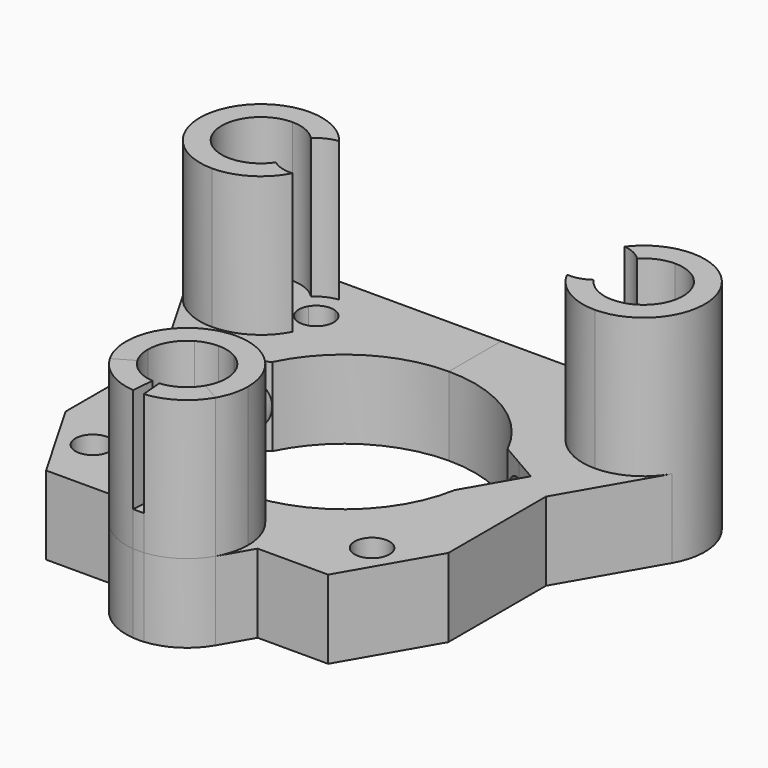
from build123d import *
from build123d import SkipClean  # not in build123d's __all__

# Parameters (mm, degrees)
F0_R     = 2
F1_DEPTH = 9
F2_DEPTH = 25
F4_DEPTH = 25
F6_DEPTH = 13


with BuildPart() as f1:
    # F0 (on Top) → F1 (new body)
    with BuildSketch(Plane.XY):
        with BuildLine():
            Line((-28.0014880557, 34.5), (-21.9393102292, 24))
            Line((-21.9393102292, 24), (-21.9393102292, 31))
            ThreePointArc((-21.9393102292, 31), (-25.4393102292, 31.9378221735), (-28.0014880557, 34.5))
        make_face()
        with BuildLine():
            Line((0, 4.5), (0, 7))
            ThreePointArc((0, 7), (-1.8117333157, 6.761480784), (-3.5, 6.0621778265))
            Line((-3.5, 6.0621778265), (-2.25, 3.897114317))
            ThreePointArc((-2.25, 3.897114317), (-1.164685703, 4.3466662183), (0, 4.5))
        make_face()
        with BuildLine():
            Line((-19.6893102292, 34.102885683), (-18.4393102292, 31.9378221735))
            ThreePointArc((-18.4393102292, 31.9378221735), (-16.8860218217, 33.1560061653), (-15.7345912365, 34.759404033))
            ThreePointArc((-15.7345912365, 34.759404033), (-17.0382696465, 34.8965993643), (-18.2150742777, 35.4741206329))
            ThreePointArc((-18.2150742777, 35.4741206329), (-18.8745190254, 34.7049954663), (-19.6893102292, 34.102885683))
        make_face()
        with BuildLine():
            Line((-3.5, 6.0621778265), (-4.7820020843, 8.282670572))
            ThreePointArc((-4.7820020843, 8.282670572), (-9.4997383801, 10.8915991321), (-12.9903810568, 15))
            Line((-12.9903810568, 15), (-15.8049636191, 13.375))
            Line((-15.8049636191, 13.375), (-8.0829037687, 0))
            Line((-8.0829037687, 0), (-7, 0))
            ThreePointArc((-7, 0), (-6.0621778265, 3.5), (-3.5, 6.0621778265))
        make_face()
        with BuildLine():
            Line((-21.9393102292, 38), (-21.9393102292, 42.5))
            ThreePointArc((-21.9393102292, 42.5), (-25.8364245462, 40.25), (-25.8364245462, 35.75))
            Line((-25.8364245462, 35.75), (-21.9393102292, 38))
        make_face()
        with BuildLine():
            Line((-2.25, 3.897114317), (-3.5, 6.0621778265))
            ThreePointArc((-3.5, 6.0621778265), (-6.0621778265, 3.5), (-7, 0))
            Line((-7, 0), (-4.5, 0))
            ThreePointArc((-4.5, 0), (-3.897114317, 2.25), (-2.25, 3.897114317))
        make_face()
        with BuildLine():
            ThreePointArc((-18.2150742777, 35.4741206329), (-17.0382696465, 34.8965993643), (-15.7345912365, 34.759404033))
            ThreePointArc((-15.7345912365, 34.759404033), (-15.3199791984, 35.7230597934), (-15.0540367364, 36.7378554248))
            ThreePointArc((-15.0540367364, 36.7378554248), (-16.3628996791, 36.5331995976), (-17.5125398242, 37.1914805006))
            ThreePointArc((-17.5125398242, 37.1914805006), (-17.7743303511, 36.296197601), (-18.2150742777, 35.4741206329))
        make_face()
        with BuildLine():
            Line((-21.9393102292, 33.5), (-21.9393102292, 38))
            Line((-21.9393102292, 38), (-25.8364245462, 35.75))
            ThreePointArc((-25.8364245462, 35.75), (-24.1893102292, 34.102885683), (-21.9393102292, 33.5))
        make_face()
        with BuildLine():
            ThreePointArc((7, 0), (4.9497474683, 4.9497474683), (0, 7))
            Line((0, 7), (0, 4.5))
            ThreePointArc((0, 4.5), (3.1819805153, 3.1819805153), (4.5, 0))
            ThreePointArc((4.5, 0), (3.3177480156, -3.0401559343), (0.3922008424, -4.4828761414))
            Line((0.3922008424, -4.4828761414), (0.6100901992, -6.9733628866))
            ThreePointArc((0.6100901992, -6.9733628866), (5.1609413577, -4.7291314533), (7, 0))
        make_face()
        with BuildLine():
            Line((-4.5, 0), (-7, 0))
            ThreePointArc((-7, 0), (-6.761480784, -1.8117333157), (-6.0621778265, -3.5))
            Line((-6.0621778265, -3.5), (-3.897114317, -2.25))
            ThreePointArc((-3.897114317, -2.25), (-4.3466662183, -1.164685703), (-4.5, 0))
        make_face()
        with BuildLine():
            ThreePointArc((4.5, 0), (3.1819805153, 3.1819805153), (0, 4.5))
            Line((0, 4.5), (0, 0))
            Line((0, 0), (0.3922008424, -4.4828761414))
            ThreePointArc((0.3922008424, -4.4828761414), (3.3177480156, -3.0401559343), (4.5, 0))
        make_face()
        with BuildLine():
            Line((-3.897114317, -2.25), (0, 0))
            Line((0, 0), (-4.5, 0))
            ThreePointArc((-4.5, 0), (-4.3466662183, -1.164685703), (-3.897114317, -2.25))
        make_face()
        with BuildLine():
            Line((-21.9393102292, 42.5), (-21.9393102292, 45))
            ThreePointArc((-21.9393102292, 45), (-28.0014880557, 41.5), (-28.0014880557, 34.5))
            Line((-28.0014880557, 34.5), (-25.8364245462, 35.75))
            ThreePointArc((-25.8364245462, 35.75), (-25.8364245462, 40.25), (-21.9393102292, 42.5))
        make_face()
        with BuildLine():
            ThreePointArc((-15.0540367364, 36.7378554248), (-15.3199791984, 35.7230597934), (-15.7345912365, 34.759404033))
            ThreePointArc((-15.7345912365, 34.759404033), (-13.256117453, 35.9439075587), (-12.25, 38.5))
            ThreePointArc((-12.25, 38.5), (-13.4802149455, 41.2772618312), (-16.3636977489, 42.2323215225))
            ThreePointArc((-16.3636977489, 42.2323215225), (-15.793812482, 41.3515455299), (-15.3619545384, 40.3954941279))
            ThreePointArc((-15.3619545384, 40.3954941279), (-14.3757938981, 39.6670280795), (-14, 38.5))
            ThreePointArc((-14, 38.5), (-14.2836191379, 37.4733370873), (-15.0540367364, 36.7378554248))
        make_face()
        with BuildLine():
            ThreePointArc((-18.6897795953, 41.1129649306), (-19.736781922, 38.1854195371), (-18.2150742777, 35.4741206329))
            ThreePointArc((-18.2150742777, 35.4741206329), (-17.7743303511, 36.296197601), (-17.5125398242, 37.1914805006))
            ThreePointArc((-17.5125398242, 37.1914805006), (-17.9929503584, 38.3322237531), (-17.7100163382, 39.5372290601))
            ThreePointArc((-17.7100163382, 39.5372290601), (-18.1178000628, 40.3761439451), (-18.6897795953, 41.1129649306))
        make_face()
        Polygon((-8.0829037687, 0), (-15.8049636191, 13.375), (-21.9393102292, 24), (-21.9393102292, 10), (-16.1658075373, 0), align=None)
        with Locations((-16, 6.5)):
            Circle(F0_R, mode=Mode.SUBTRACT)
        with BuildLine():
            ThreePointArc((-21.9393102292, 33.5), (-20.7746245262, 33.6533337817), (-19.6893102292, 34.102885683))
            Line((-19.6893102292, 34.102885683), (-21.9393102292, 38))
            Line((-21.9393102292, 38), (-21.9393102292, 33.5))
        make_face()
        with BuildLine():
            ThreePointArc((-16.3636977489, 42.2323215225), (-18.8269357866, 44.2700179688), (-21.9393102292, 45))
            Line((-21.9393102292, 45), (-21.9393102292, 42.5))
            ThreePointArc((-21.9393102292, 42.5), (-20.1727234337, 42.1387402786), (-18.6897795953, 41.1129649306))
            ThreePointArc((-18.6897795953, 41.1129649306), (-17.6260906395, 41.8791018381), (-16.3636977489, 42.2323215225))
        make_face()
        with BuildLine():
            Line((0, 0), (0, 4.5))
            ThreePointArc((0, 4.5), (-1.164685703, 4.3466662183), (-2.25, 3.897114317))
            Line((-2.25, 3.897114317), (0, 0))
        make_face()
        with BuildLine():
            ThreePointArc((-13.488307945, 29.0624346688), (-7.9549820857, 35.2168494532), (0, 37.5))
            Line((0, 37.5), (0, 38))
            Line((0, 38), (0, 45))
            Line((0, 45), (-21.9393102292, 45))
            ThreePointArc((-21.9393102292, 45), (-18.8269357866, 44.2700179688), (-16.3636977489, 42.2323215225))
            ThreePointArc((-16.3636977489, 42.2323215225), (-13.4802149455, 41.2772618312), (-12.25, 38.5))
            ThreePointArc((-12.25, 38.5), (-13.256117453, 35.9439075587), (-15.7345912365, 34.759404033))
            ThreePointArc((-15.7345912365, 34.759404033), (-16.8860218217, 33.1560061653), (-18.4393102292, 31.9378221735))
            Line((-18.4393102292, 31.9378221735), (-15.9564803457, 27.6374346688))
            Line((-15.9564803457, 27.6374346688), (-13.488307945, 29.0624346688))
        make_face()
        with BuildLine():
            Line((-21.9393102292, 38), (-19.6893102292, 34.102885683))
            ThreePointArc((-19.6893102292, 34.102885683), (-18.8745190254, 34.7049954663), (-18.2150742777, 35.4741206329))
            ThreePointArc((-18.2150742777, 35.4741206329), (-19.736781922, 38.1854195371), (-18.6897795953, 41.1129649306))
            ThreePointArc((-18.6897795953, 41.1129649306), (-20.1727234337, 42.1387402786), (-21.9393102292, 42.5))
            Line((-21.9393102292, 42.5), (-21.9393102292, 38))
        make_face()
        with BuildLine():
            ThreePointArc((-21.9393102292, 31), (-20.1275769135, 31.238519216), (-18.4393102292, 31.9378221735))
            Line((-18.4393102292, 31.9378221735), (-19.6893102292, 34.102885683))
            ThreePointArc((-19.6893102292, 34.102885683), (-20.7746245262, 33.6533337817), (-21.9393102292, 33.5))
            Line((-21.9393102292, 33.5), (-21.9393102292, 31))
        make_face()
        with BuildLine():
            Line((-15.8049636191, 13.375), (-12.9903810568, 15))
            ThreePointArc((-12.9903810568, 15), (-14.0930796876, 17.3633566487), (-14.7697665097, 19.8819860108))
            Line((-14.7697665097, 19.8819860108), (-18.4246527465, 26.2124346688))
            Line((-18.4246527465, 26.2124346688), (-15.9564803457, 27.6374346688))
            Line((-15.9564803457, 27.6374346688), (-18.4393102292, 31.9378221735))
            ThreePointArc((-18.4393102292, 31.9378221735), (-20.1275769135, 31.238519216), (-21.9393102292, 31))
            Line((-21.9393102292, 31), (-21.9393102292, 24))
            Line((-21.9393102292, 24), (-15.8049636191, 13.375))
        make_face()
        with BuildLine():
            Line((0, 7), (0, 7.5))
            ThreePointArc((0, 7.5), (-2.4228143325, 7.696960761), (-4.7820020843, 8.282670572))
            Line((-4.7820020843, 8.282670572), (-3.5, 6.0621778265))
            ThreePointArc((-3.5, 6.0621778265), (-1.8117333157, 6.761480784), (0, 7))
        make_face()
        with BuildLine():
            ThreePointArc((-15.3619545384, 40.3954941279), (-15.793812482, 41.3515455299), (-16.3636977489, 42.2323215225))
            ThreePointArc((-16.3636977489, 42.2323215225), (-17.6260906395, 41.8791018381), (-18.6897795953, 41.1129649306))
            ThreePointArc((-18.6897795953, 41.1129649306), (-18.1178000628, 40.3761439451), (-17.7100163382, 39.5372290601))
            ThreePointArc((-17.7100163382, 39.5372290601), (-16.6866113324, 40.3784474649), (-15.3619545384, 40.3954941279))
        make_face()
        with BuildLine():
            Line((-4.5, 0), (0, 0))
            Line((0, 0), (-2.25, 3.897114317))
            ThreePointArc((-2.25, 3.897114317), (-3.897114317, 2.25), (-4.5, 0))
        make_face()
        with BuildLine():
            ThreePointArc((-28.0014880557, 34.5), (-25.4393102292, 31.9378221735), (-21.9393102292, 31))
            Line((-21.9393102292, 31), (-21.9393102292, 33.5))
            ThreePointArc((-21.9393102292, 33.5), (-24.1893102292, 34.102885683), (-25.8364245462, 35.75))
            Line((-25.8364245462, 35.75), (-28.0014880557, 34.5))
        make_face()
        with BuildLine():
            ThreePointArc((-6.0621778265, -3.5), (-6.761480784, -1.8117333157), (-7, 0))
            Line((-7, 0), (-8.0829037687, 0))
            Line((-8.0829037687, 0), (-6.0621778265, -3.5))
        make_face()
        with BuildLine():
            Line((-0.3922008424, -4.4828761414), (0, 0))
            Line((0, 0), (-3.897114317, -2.25))
            ThreePointArc((-3.897114317, -2.25), (-2.4178482376, -3.7952615062), (-0.3922008424, -4.4828761414))
        make_face()
        with BuildLine():
            ThreePointArc((-0.3922008424, -4.4828761414), (-2.4178482376, -3.7952615062), (-3.897114317, -2.25))
            Line((-3.897114317, -2.25), (-6.0621778265, -3.5))
            ThreePointArc((-6.0621778265, -3.5), (-3.7610972584, -5.9037401207), (-0.6100901992, -6.9733628866))
            Line((-0.6100901992, -6.9733628866), (-0.3922008424, -4.4828761414))
        make_face()
        with BuildLine():
            ThreePointArc((-0.6100901992, -6.9733628866), (0, -7), (0.6100901992, -6.9733628866))
            Line((0.6100901992, -6.9733628866), (0.3922008424, -4.4828761414))
            ThreePointArc((0.3922008424, -4.4828761414), (0, -4.5), (-0.3922008424, -4.4828761414))
            Line((-0.3922008424, -4.4828761414), (-0.6100901992, -6.9733628866))
        make_face()
        with BuildLine():
            Line((0.3922008424, -4.4828761414), (0, 0))
            Line((0, 0), (-0.3922008424, -4.4828761414))
            ThreePointArc((-0.3922008424, -4.4828761414), (0, -4.5), (0.3922008424, -4.4828761414))
        make_face()
    extrude(amount=F1_DEPTH)

    # F0 (on Top) → F2 (join)
    with BuildSketch(Plane.XY):
        with BuildLine():
            ThreePointArc((7, 0), (4.9497474683, 4.9497474683), (0, 7))
            Line((0, 7), (0, 4.5))
            ThreePointArc((0, 4.5), (3.1819805153, 3.1819805153), (4.5, 0))
            ThreePointArc((4.5, 0), (3.3177480156, -3.0401559343), (0.3922008424, -4.4828761414))
            Line((0.3922008424, -4.4828761414), (0.6100901992, -6.9733628866))
            ThreePointArc((0.6100901992, -6.9733628866), (5.1609413577, -4.7291314533), (7, 0))
        make_face()
        with BuildLine():
            Line((-2.25, 3.897114317), (-3.5, 6.0621778265))
            ThreePointArc((-3.5, 6.0621778265), (-6.0621778265, 3.5), (-7, 0))
            Line((-7, 0), (-4.5, 0))
            ThreePointArc((-4.5, 0), (-3.897114317, 2.25), (-2.25, 3.897114317))
        make_face()
        with BuildLine():
            Line((-19.6893102292, 34.102885683), (-18.4393102292, 31.9378221735))
            ThreePointArc((-18.4393102292, 31.9378221735), (-16.8860218217, 33.1560061653), (-15.7345912365, 34.759404033))
            ThreePointArc((-15.7345912365, 34.759404033), (-17.0382696465, 34.8965993643), (-18.2150742777, 35.4741206329))
            ThreePointArc((-18.2150742777, 35.4741206329), (-18.8745190254, 34.7049954663), (-19.6893102292, 34.102885683))
        make_face()
        with BuildLine():
            ThreePointArc((-21.9393102292, 31), (-20.1275769135, 31.238519216), (-18.4393102292, 31.9378221735))
            Line((-18.4393102292, 31.9378221735), (-19.6893102292, 34.102885683))
            ThreePointArc((-19.6893102292, 34.102885683), (-20.7746245262, 33.6533337817), (-21.9393102292, 33.5))
            Line((-21.9393102292, 33.5), (-21.9393102292, 31))
        make_face()
        with BuildLine():
            ThreePointArc((-28.0014880557, 34.5), (-25.4393102292, 31.9378221735), (-21.9393102292, 31))
            Line((-21.9393102292, 31), (-21.9393102292, 33.5))
            ThreePointArc((-21.9393102292, 33.5), (-24.1893102292, 34.102885683), (-25.8364245462, 35.75))
            Line((-25.8364245462, 35.75), (-28.0014880557, 34.5))
        make_face()
        with BuildLine():
            Line((-21.9393102292, 42.5), (-21.9393102292, 45))
            ThreePointArc((-21.9393102292, 45), (-28.0014880557, 41.5), (-28.0014880557, 34.5))
            Line((-28.0014880557, 34.5), (-25.8364245462, 35.75))
            ThreePointArc((-25.8364245462, 35.75), (-25.8364245462, 40.25), (-21.9393102292, 42.5))
        make_face()
        with BuildLine():
            ThreePointArc((-16.3636977489, 42.2323215225), (-18.8269357866, 44.2700179688), (-21.9393102292, 45))
            Line((-21.9393102292, 45), (-21.9393102292, 42.5))
            ThreePointArc((-21.9393102292, 42.5), (-20.1727234337, 42.1387402786), (-18.6897795953, 41.1129649306))
            ThreePointArc((-18.6897795953, 41.1129649306), (-17.6260906395, 41.8791018381), (-16.3636977489, 42.2323215225))
        make_face()
        with BuildLine():
            Line((-4.5, 0), (-7, 0))
            ThreePointArc((-7, 0), (-6.761480784, -1.8117333157), (-6.0621778265, -3.5))
            Line((-6.0621778265, -3.5), (-3.897114317, -2.25))
            ThreePointArc((-3.897114317, -2.25), (-4.3466662183, -1.164685703), (-4.5, 0))
        make_face()
        with BuildLine():
            Line((0, 4.5), (0, 7))
            ThreePointArc((0, 7), (-1.8117333157, 6.761480784), (-3.5, 6.0621778265))
            Line((-3.5, 6.0621778265), (-2.25, 3.897114317))
            ThreePointArc((-2.25, 3.897114317), (-1.164685703, 4.3466662183), (0, 4.5))
        make_face()
    extrude(amount=F2_DEPTH)

    # F3 (on face) → F4 (cut)
    with BuildSketch(Plane(origin=(-15.9564803457, 27.6374346688, 0), x_dir=(0.8660254038, 0.5, 0), z_dir=(0.5, -0.8660254038, 0))):
        with BuildLine():
            ThreePointArc((2.85, 4.5), (2.0152543264, 6.5152543264), (0, 7.35))
            Line((0, 7.35), (0, 1.65))
            ThreePointArc((0, 1.65), (2.0152543264, 2.4847456736), (2.85, 4.5))
        make_face()
        with BuildLine():
            Line((0, 1.65), (0, 7.35))
            ThreePointArc((0, 7.35), (-2.0152543264, 6.5152543264), (-2.85, 4.5))
            ThreePointArc((-2.85, 4.5), (-2.0152543264, 2.4847456736), (0, 1.65))
        make_face()
    extrude(amount=-F4_DEPTH, mode=Mode.SUBTRACT)

    # F5: F1 across plane


with BuildPart() as f1_1:
    add(f1.part, clean=False)
    with SkipClean():  # cleaning this boolean's faces spoils the solid; the shape is the same uncleaned
        add(f1.part.mirror(Plane.YZ), clean=False)

    # F0 (on Top) → F6 (join)
    with BuildSketch(Plane.XY):
        with BuildLine():
            Line((0.3922008424, -4.4828761414), (0, 0))
            Line((0, 0), (-0.3922008424, -4.4828761414))
            ThreePointArc((-0.3922008424, -4.4828761414), (0, -4.5), (0.3922008424, -4.4828761414))
        make_face()
        with BuildLine():
            ThreePointArc((-0.6100901992, -6.9733628866), (0, -7), (0.6100901992, -6.9733628866))
            Line((0.6100901992, -6.9733628866), (0.3922008424, -4.4828761414))
            ThreePointArc((0.3922008424, -4.4828761414), (0, -4.5), (-0.3922008424, -4.4828761414))
            Line((-0.3922008424, -4.4828761414), (-0.6100901992, -6.9733628866))
        make_face()
        with BuildLine():
            Line((-0.3922008424, -4.4828761414), (0, 0))
            Line((0, 0), (-3.897114317, -2.25))
            ThreePointArc((-3.897114317, -2.25), (-2.4178482376, -3.7952615062), (-0.3922008424, -4.4828761414))
        make_face()
        with BuildLine():
            ThreePointArc((4.5, 0), (3.1819805153, 3.1819805153), (0, 4.5))
            Line((0, 4.5), (0, 0))
            Line((0, 0), (0.3922008424, -4.4828761414))
            ThreePointArc((0.3922008424, -4.4828761414), (3.3177480156, -3.0401559343), (4.5, 0))
        make_face()
        with BuildLine():
            Line((0, 0), (0, 4.5))
            ThreePointArc((0, 4.5), (-1.164685703, 4.3466662183), (-2.25, 3.897114317))
            Line((-2.25, 3.897114317), (0, 0))
        make_face()
        with BuildLine():
            Line((-4.5, 0), (0, 0))
            Line((0, 0), (-2.25, 3.897114317))
            ThreePointArc((-2.25, 3.897114317), (-3.897114317, 2.25), (-4.5, 0))
        make_face()
        with BuildLine():
            Line((-3.897114317, -2.25), (0, 0))
            Line((0, 0), (-4.5, 0))
            ThreePointArc((-4.5, 0), (-4.3466662183, -1.164685703), (-3.897114317, -2.25))
        make_face()
    with SkipClean():  # cleaning this boolean's faces spoils the solid; the shape is the same uncleaned
        extrude(amount=F6_DEPTH)


solid = f1_1.part
